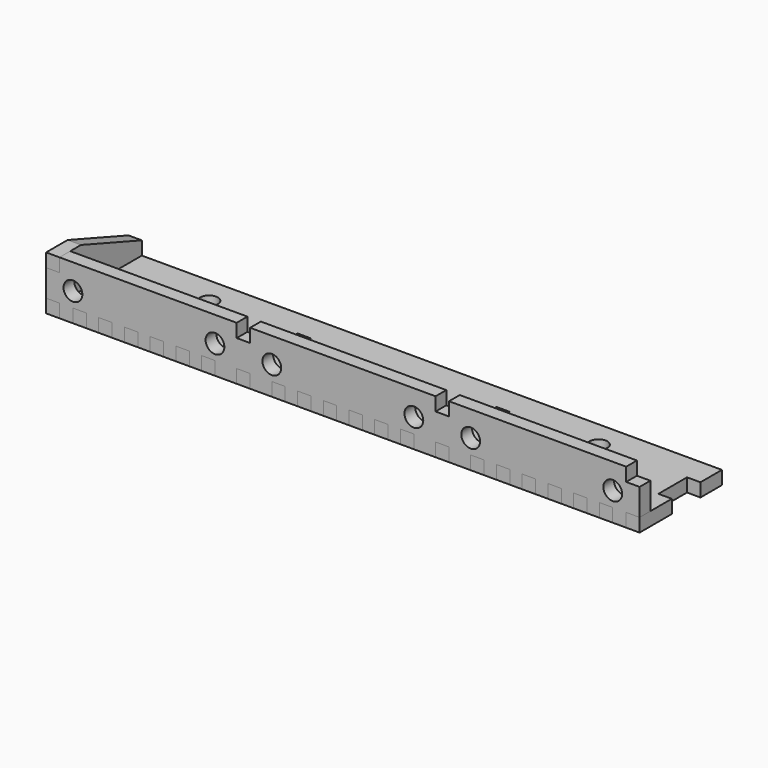
from build123d import *

# Parameters (mm, degrees)
F0_W      = 132.65
F0_H      = 12
F0_R      = 2.1
F3_DEPTH  = 3
F1_W      = 3
F1_H      = 3
F4_DEPTH  = 3.001
F2_W      = 132.65
F2_H      = 3
F5_DEPTH  = 20
F6_DEPTH  = 3
F7_W      = 3
F7_H      = 8
F8_DEPTH  = 3.001
F9_W      = 3
F9_H      = 3
F10_DEPTH = 3.001
F11_R     = 2
F13_DEPTH = 3.001
F14_DEPTH = 3


# Not quite as in the source:
# - a feature names something its author has since deleted; it is built from what else it names


with BuildPart() as f3:
    # F0 (on Front) → F3 (new body)
    with BuildSketch(Plane.XZ):
        with Locations((66.325, 6)):
            Rectangle(F0_W, F0_H)
        with Locations((6, 6.35)):
            Circle(F0_R, mode=Mode.SUBTRACT)
        with Locations((37.75, 6.35)):
            Circle(F0_R, mode=Mode.SUBTRACT)
        with Locations((50.45, 6.35)):
            Circle(F0_R, mode=Mode.SUBTRACT)
        with Locations((82.2, 6.35)):
            Circle(F0_R, mode=Mode.SUBTRACT)
        with Locations((94.9, 6.35)):
            Circle(F0_R, mode=Mode.SUBTRACT)
        with Locations((126.65, 6.35)):
            Circle(F0_R, mode=Mode.SUBTRACT)
    extrude(amount=F3_DEPTH)

    # F1 (on face) → F4 (cut, through all)
    with BuildSketch(Plane.XZ):
        with Locations((1.5, 1.5)):
            Rectangle(F1_W, F1_H)
        with Locations((7.5, 1.5)):
            Rectangle(F1_W, F1_H)
        with Locations((13.25, 1.5)):
            Rectangle(F1_W, F1_H)
        with Locations((19, 1.5)):
            Rectangle(F1_W, F1_H)
        with Locations((24.75, 1.5)):
            Rectangle(F1_W, F1_H)
        with Locations((30.5, 1.5)):
            Rectangle(F1_W, F1_H)
        with Locations((36.25, 1.5)):
            Rectangle(F1_W, F1_H)
        with Locations((44.1, 1.5)):
            Rectangle(F1_W, F1_H)
        with Locations((51.95, 1.5)):
            Rectangle(F1_W, F1_H)
        with Locations((57.7, 1.5)):
            Rectangle(F1_W, F1_H)
        with Locations((63.45, 1.5)):
            Rectangle(F1_W, F1_H)
        with Locations((69.2, 1.5)):
            Rectangle(F1_W, F1_H)
        with Locations((74.95, 1.5)):
            Rectangle(F1_W, F1_H)
        with Locations((80.7, 1.5)):
            Rectangle(F1_W, F1_H)
        with Locations((88.55, 1.5)):
            Rectangle(F1_W, F1_H)
        with Locations((96.4, 1.5)):
            Rectangle(F1_W, F1_H)
        with Locations((102.15, 1.5)):
            Rectangle(F1_W, F1_H)
        with Locations((107.9, 1.5)):
            Rectangle(F1_W, F1_H)
        with Locations((113.65, 1.5)):
            Rectangle(F1_W, F1_H)
        with Locations((119.4, 1.5)):
            Rectangle(F1_W, F1_H)
        with Locations((125.15, 1.5)):
            Rectangle(F1_W, F1_H)
    extrude(amount=F4_DEPTH, mode=Mode.SUBTRACT)

    # F9 (on face) → F10 (cut, through all)
    with BuildSketch(Plane.XZ):
        with Locations((88.55, 10.5)):
            Rectangle(F9_W, F9_H)
        with Locations((131.15, 10.5)):
            Rectangle(F9_W, F9_H)
        with Locations((44.1, 10.5)):
            Rectangle(F9_W, F9_H)
        with Locations((1.5, 10.5)):
            Rectangle(F9_W, F9_H)
    extrude(amount=F10_DEPTH, mode=Mode.SUBTRACT)


with BuildPart() as f5:
    # F2 (on Front) → F5 (new body)
    with BuildSketch(Plane.XZ):
        with Locations((66.325, 1.5)):
            Rectangle(F2_W, F2_H)
    extrude(amount=-F5_DEPTH)

    # F1 (on face) → F6 (join)
    with BuildSketch(Plane.XZ):
        with Locations((125.15, 1.5)):
            Rectangle(F1_W, F1_H)
        with Locations((119.4, 1.5)):
            Rectangle(F1_W, F1_H)
        with Locations((113.65, 1.5)):
            Rectangle(F1_W, F1_H)
        with Locations((107.9, 1.5)):
            Rectangle(F1_W, F1_H)
        with Locations((102.15, 1.5)):
            Rectangle(F1_W, F1_H)
        with Locations((96.4, 1.5)):
            Rectangle(F1_W, F1_H)
        with Locations((88.55, 1.5)):
            Rectangle(F1_W, F1_H)
        with Locations((80.7, 1.5)):
            Rectangle(F1_W, F1_H)
        with Locations((74.95, 1.5)):
            Rectangle(F1_W, F1_H)
        with Locations((69.2, 1.5)):
            Rectangle(F1_W, F1_H)
        with Locations((63.45, 1.5)):
            Rectangle(F1_W, F1_H)
        with Locations((57.7, 1.5)):
            Rectangle(F1_W, F1_H)
        with Locations((51.95, 1.5)):
            Rectangle(F1_W, F1_H)
        with Locations((44.1, 1.5)):
            Rectangle(F1_W, F1_H)
        with Locations((36.25, 1.5)):
            Rectangle(F1_W, F1_H)
        with Locations((30.5, 1.5)):
            Rectangle(F1_W, F1_H)
        with Locations((24.75, 1.5)):
            Rectangle(F1_W, F1_H)
        with Locations((19, 1.5)):
            Rectangle(F1_W, F1_H)
        with Locations((13.25, 1.5)):
            Rectangle(F1_W, F1_H)
        with Locations((7.5, 1.5)):
            Rectangle(F1_W, F1_H)
        with Locations((1.5, 1.5)):
            Rectangle(F1_W, F1_H)
        with Locations((131.15, 1.5)):
            Rectangle(F1_W, F1_H)
    extrude(amount=F6_DEPTH)

    # F7 (on face) → F8 (cut, through all)
    with BuildSketch(Plane.XY.offset(3)):
        with Locations((131.15, 10)):
            Rectangle(F7_W, F7_H)
        with Locations((44.1, 10)):
            Rectangle(F7_W, F7_H)
        with Locations((1.5, 10)):
            Rectangle(F7_W, F7_H)
        with Locations((88.55, 10)):
            Rectangle(F7_W, F7_H)
    extrude(amount=-F8_DEPTH, mode=Mode.SUBTRACT)

    # F11 (on face) → F13 (cut, through all)
    with BuildSketch(Plane.XY.offset(3)):
        with Locations((66.325, 6)):
            Circle(F11_R)
        with Locations((109.85, 14)):
            Circle(F11_R)
        with Locations((22.8, 14)):
            Circle(F11_R)
    extrude(amount=-F13_DEPTH, mode=Mode.SUBTRACT)


with BuildPart() as f14:
    # F12 (on face) → F14 (new body)
    with BuildSketch(Plane(origin=(0, 0, 0), x_dir=(0, -1, 0), z_dir=(-1, 0, 0))):
        Polygon((-20, 6), (-20, 3), (-14, 3), (-14, 0), (-6, 0), (-6, 3), (0, 3), (0, 9), (3, 9), (3, 12), (-3, 12), align=None)
    extrude(amount=-F14_DEPTH)


solid = Compound([f3.part, f5.part, f14.part])
